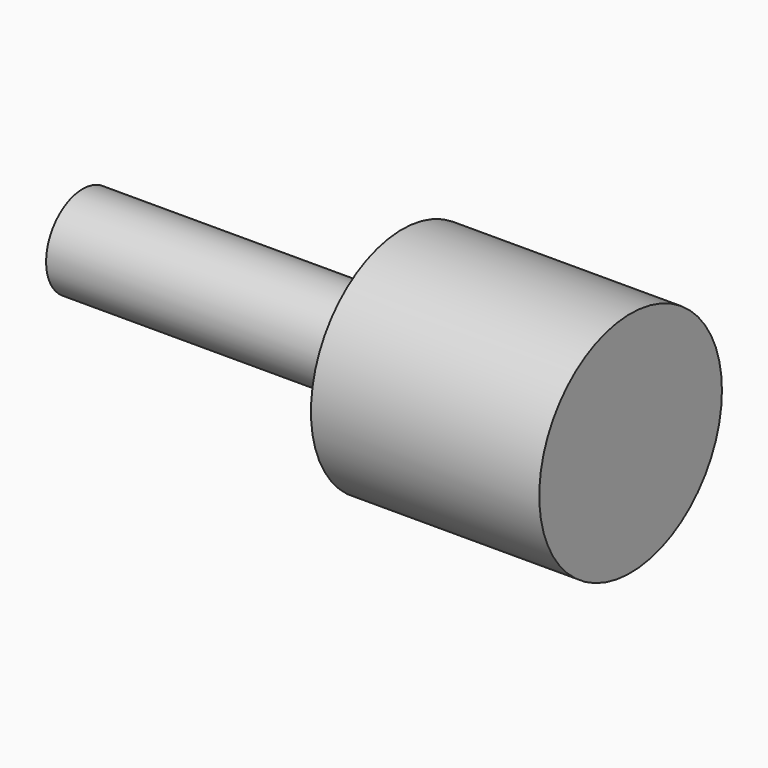
from build123d import *

# Parameters (mm, degrees)
F0_R     = 15.875
F1_DEPTH = 15.875
F6_R     = 6.35
F7_DEPTH = 44.45


# Not quite as in the source:
# - the program builds the solid bodies; features that only make, move or delete a surface that nothing else refers to are left out


with BuildPart() as f1:
    # F0 (on Right) → F1 (new body, symmetric)
    with BuildSketch(Plane.YZ):
        Circle(F0_R)
    extrude(amount=F1_DEPTH, both=True)

    # F6 (on face) → F7 (join)
    with BuildSketch(Plane(origin=(-15.875, 0, 0), x_dir=(0, -1, 0), z_dir=(-1, 0, 0))):
        Circle(F6_R)
    extrude(amount=F7_DEPTH)


solid = f1.part
